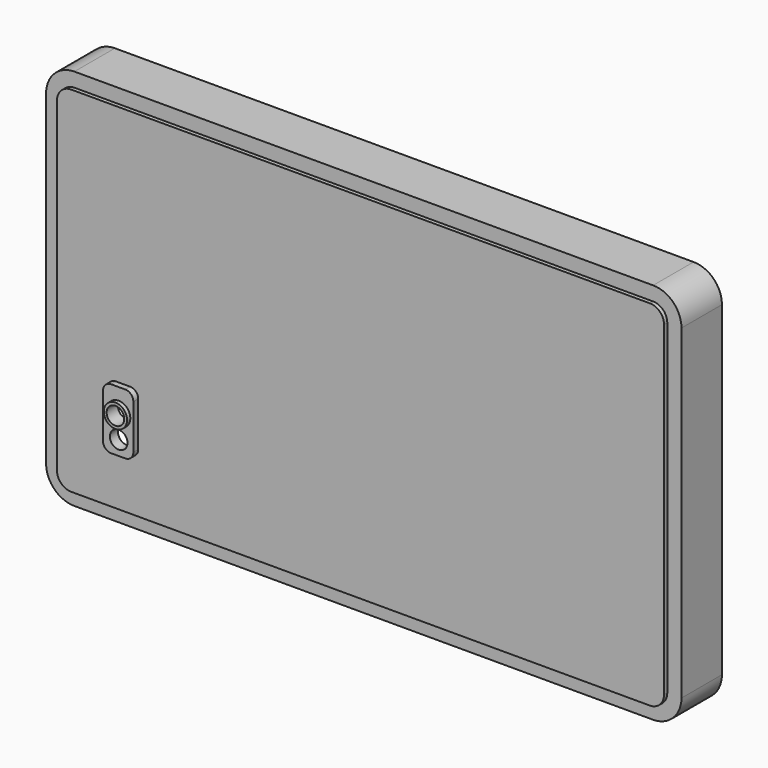
from build123d import *

# Parameters (mm, degrees)
F1_DEPTH = 25
F2_DEPTH = 2
F0_R     = 4.348998023
F0_R_2   = 5.7489946485
F3_DEPTH = 5
F4_DEPTH = 7


with BuildPart() as f1:
    # F0 (on Front) → F1 (new body)
    with BuildSketch(Plane.XZ):
        with BuildLine():
            Line((145.9706694186, 87.1744155884), (-140.0293305814, 87.1744155884))
            ThreePointArc((-140.0293305814, 87.1744155884), (-149.9288249466, 83.0739107617), (-154.0293297732, 73.1744163966))
            Line((-154.0293297732, 73.1744163966), (-154.0293297732, -87.8255836034))
            ThreePointArc((-154.0293297732, -87.8255836034), (-149.9288249466, -97.7250779685), (-140.0293305814, -101.8255827952))
            Line((-140.0293305814, -101.8255827952), (145.9706694186, -101.8255827952))
            ThreePointArc((145.9706694186, -101.8255827952), (155.8701637837, -97.7250779685), (159.9706686104, -87.8255836034))
            Line((159.9706686104, -87.8255836034), (159.9706686104, 73.1744163966))
            ThreePointArc((159.9706686104, 73.1744163966), (155.8701637837, 83.0739107617), (145.9706694186, 87.1744155884))
        make_face()
        with BuildLine():
            ThreePointArc((-147.0293305814, 73.1744163966), (-144.9790780497, 78.1241638649), (-140.0293305814, 80.1744163966))
            Line((-140.0293305814, 80.1744163966), (145.9706694186, 80.1744163966))
            ThreePointArc((145.9706694186, 80.1744163966), (150.9204168869, 78.1241638649), (152.9706694186, 73.1744163966))
            Line((152.9706694186, 73.1744163966), (152.9706694186, -87.8255836034))
            ThreePointArc((152.9706694186, -87.8255836034), (150.9204168869, -92.7753310717), (145.9706694186, -94.8255836034))
            Line((145.9706694186, -94.8255836034), (-140.0293305814, -94.8255836034))
            ThreePointArc((-140.0293305814, -94.8255836034), (-144.9790780497, -92.7753310717), (-147.0293305814, -87.8255836034))
            Line((-147.0293305814, -87.8255836034), (-147.0293305814, 73.1744163966))
        make_face(mode=Mode.SUBTRACT)
    extrude(amount=-F1_DEPTH)


with BuildPart() as f2:
    # F0 (on Front) → F2 (new body)
    with BuildSketch(Plane.XZ):
        with BuildLine():
            Line((145.9706694186, 80.1744163966), (-140.0293305814, 80.1744163966))
            ThreePointArc((-140.0293305814, 80.1744163966), (-144.9790780497, 78.1241638649), (-147.0293305814, 73.1744163966))
            Line((-147.0293305814, 73.1744163966), (-147.0293305814, -87.8255836034))
            ThreePointArc((-147.0293305814, -87.8255836034), (-144.9790780497, -92.7753310717), (-140.0293305814, -94.8255836034))
            Line((-140.0293305814, -94.8255836034), (145.9706694186, -94.8255836034))
            ThreePointArc((145.9706694186, -94.8255836034), (150.9204168869, -92.7753310717), (152.9706694186, -87.8255836034))
            Line((152.9706694186, -87.8255836034), (152.9706694186, 73.1744163966))
            ThreePointArc((152.9706694186, 73.1744163966), (150.9204168869, 78.1241638649), (145.9706694186, 80.1744163966))
        make_face()
        with BuildLine():
            ThreePointArc((-121.900819242, -43.6237730914), (-120.7292463667, -40.7953459667), (-117.900819242, -39.6237730914))
            Line((-117.900819242, -39.6237730914), (-110.900819242, -39.6237730914))
            ThreePointArc((-110.900819242, -39.6237730914), (-108.0723921173, -40.7953459667), (-106.900819242, -43.6237730914))
            Line((-106.900819242, -43.6237730914), (-106.900819242, -65.6237730914))
            ThreePointArc((-106.900819242, -65.6237730914), (-108.0723921173, -68.4522002162), (-110.900819242, -69.6237730914))
            Line((-110.900819242, -69.6237730914), (-117.900819242, -69.6237730914))
            ThreePointArc((-117.900819242, -69.6237730914), (-120.7292463667, -68.4522002162), (-121.900819242, -65.6237730914))
            Line((-121.900819242, -65.6237730914), (-121.900819242, -43.6237730914))
        make_face(mode=Mode.SUBTRACT)
    extrude(amount=F2_DEPTH)


with BuildPart() as f3:
    # F0 (on Front) → F3 (new body)
    with BuildSketch(Plane.XZ):
        with BuildLine():
            Line((-110.900819242, -39.6237730914), (-117.900819242, -39.6237730914))
            ThreePointArc((-117.900819242, -39.6237730914), (-120.7292463667, -40.7953459667), (-121.900819242, -43.6237730914))
            Line((-121.900819242, -43.6237730914), (-121.900819242, -65.6237730914))
            ThreePointArc((-121.900819242, -65.6237730914), (-120.7292463667, -68.4522002162), (-117.900819242, -69.6237730914))
            Line((-117.900819242, -69.6237730914), (-110.900819242, -69.6237730914))
            ThreePointArc((-110.900819242, -69.6237730914), (-108.0723921173, -68.4522002162), (-106.900819242, -65.6237730914))
            Line((-106.900819242, -65.6237730914), (-106.900819242, -43.6237730914))
            ThreePointArc((-106.900819242, -43.6237730914), (-108.0723921173, -40.7953459667), (-110.900819242, -39.6237730914))
        make_face()
        with Locations((-114.151455462, -62.5361315906)):
            Circle(F0_R, mode=Mode.SUBTRACT)
        with Locations((-114.151455462, -51.313970238)):
            Circle(F0_R_2, mode=Mode.SUBTRACT)
        with Locations((-114.151455462, -51.313970238)):
            Circle(F0_R_2)
        with Locations((-114.151455462, -51.313970238)):
            Circle(F0_R, mode=Mode.SUBTRACT)
    extrude(amount=F3_DEPTH)


with BuildPart() as f4:
    # F0 (on Front) → F4 (new body)
    with BuildSketch(Plane.XZ):
        with Locations((-114.151455462, -51.313970238)):
            Circle(F0_R_2)
        with Locations((-114.151455462, -51.313970238)):
            Circle(F0_R, mode=Mode.SUBTRACT)
    extrude(amount=F4_DEPTH)


solid = Compound([f1.part, f2.part, f3.part, f4.part])
